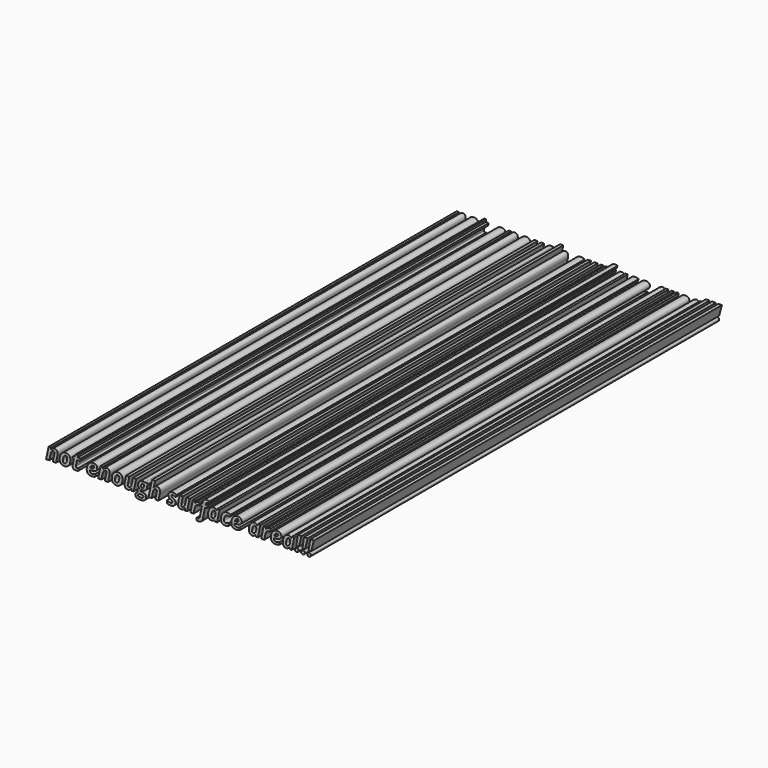
from build123d import *

# Parameters (mm, degrees)
F0_TEXT_SIZE = 1072.5280476941
F1_DEPTH     = 25374.6


# Not quite as in the source:
# - Text() gives the source's letters only with a copy of the font that has no kerning and outlines rounded to 1/6400 em; it was checked with that copy


with BuildPart() as f1:
    # F0 (on Front) → F1 (new body)
    with BuildSketch(Plane.XZ):
        with Locations((-137.2931450605, -147.3623216152)):
            Text('not enough surface area!!!', F0_TEXT_SIZE, font='Open Sans', font_style=FontStyle.BOLDITALIC, text_align=(TextAlign.LEFT, TextAlign.BOTTOM))
    extrude(amount=F1_DEPTH)


solid = f1.part
